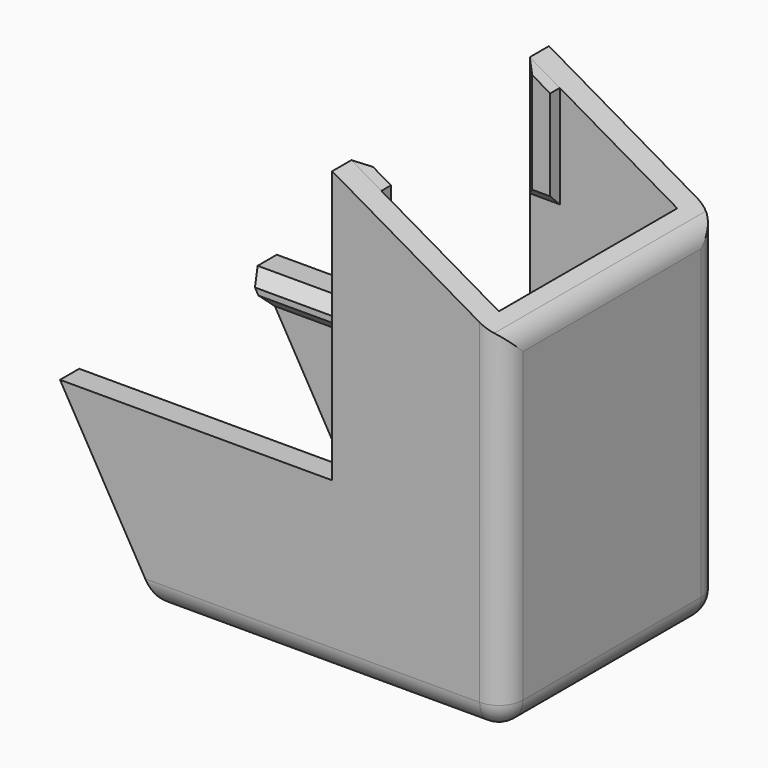
from build123d import *

# Parameters (mm, degrees)
F4_W      = 35
F4_H      = 18.6
F5_DEPTH  = 2
F4_W_2    = 2
F4_H_2    = 2
F6_DEPTH  = 37
F7_DEPTH  = 14.3
F8_W      = 2
F8_H      = 22.7
F9_DEPTH  = 12.3
F11_DEPTH = 22.6
F12_R     = 2
F14_DEPTH = 1
F15_SIZE  = 0.99999
F17_DEPTH = 1
F18_SIZE  = 0.99999


# Not quite as in the source:
# - a fillet or chamfer is up to 0.001 mm smaller than in the source, because OpenCascade refuses the exact size


with BuildPart() as f5:
    # F4 (on Top) → F5 (new body)
    with BuildSketch(Plane.XY):
        with Locations((17.5, -11.3)):
            Rectangle(F4_W, F4_H)
    extrude(amount=F5_DEPTH)

    # F4 (on Top) → F6 (join)
    with BuildSketch(Plane.XY):
        with Locations((36, -11.3)):
            Rectangle(F4_W_2, F4_H)
        with Locations((36, -21.6)):
            Rectangle(F4_W_2, F4_H_2)
        with Locations((36, -1)):
            Rectangle(F4_W_2, F4_H_2)
    extrude(amount=F6_DEPTH)

    # F4 (on Top) → F7 (join)
    with BuildSketch(Plane.XY):
        with Locations((17.5, -1)):
            Rectangle(F4_W, F4_H_2)
        with Locations((17.5, -21.6)):
            Rectangle(F4_W, F4_H_2)
    extrude(amount=F7_DEPTH)

    # F8 (on face) → F9 (join)
    with BuildSketch(Plane(origin=(35, 0, 0), x_dir=(0, -1, 0), z_dir=(-1, 0, 0))):
        with Locations((1, 25.65)):
            Rectangle(F8_W, F8_H)
        with Locations((21.6, 25.65)):
            Rectangle(F8_W, F8_H)
    extrude(amount=F9_DEPTH)

    # F10 (on face) → F11 (cut)
    with BuildSketch(Plane.XZ.offset(22.6)):
        Polygon((8.2561088494, 0), (0, 14.3), (0, 0), align=None)
        Polygon((37, 37), (22.7, 37), (37, 28.7438911506), align=None)
    extrude(amount=-F11_DEPTH, mode=Mode.SUBTRACT)

    # F12
    f12_edges = [f5.edges().sort_by_distance(p)[0] for p in [
        (37, -11.3, 0),
        (22.628054, -22.6, 0),
        (37, -22.6, 14.371946),
        (37, 0, 14.371946),
        (22.628054, 0, 0),
        (8.256109, -11.3, 0),
        (37, -11.3, 28.743891),
    ]]
    fillet(f12_edges, radius=F12_R)

    # F13 (on face) → F14 (join)
    with BuildSketch(Plane.XZ.offset(2)):
        Polygon((25.2, 35.556624327), (22.7, 37), (22.7, 27), (25.2, 27), align=None)
        Polygon((10, 11.8), (10, 14.3), (0, 14.3), (1.443375673, 11.8), align=None)
    extrude(amount=F14_DEPTH)

    # F15 (size 1 in the source; OpenCascade refuses exactly that, so slightly less here)
    f15_edges = [f5.edges().sort_by_distance(p)[0] for p in [
        (23.95, -3, 27),
        (5.721688, -3, 11.8),
        (22.7, -3, 32),
        (5, -3, 14.3),
    ]]
    chamfer(f15_edges, length=F15_SIZE)

    # F16 (on face) → F17 (join)
    with BuildSketch(Plane(origin=(0, -20.6, 0), x_dir=(-1, 0, 0), z_dir=(0, 1, 0))):
        Polygon((-22.7, 27), (-22.7, 37), (-25.2, 35.556624327), (-25.2, 27), align=None)
        Polygon((0, 14.3), (-10, 14.3), (-10, 11.8), (-1.443375673, 11.8), align=None)
    extrude(amount=F17_DEPTH)

    # F18 (size 1 in the source; OpenCascade refuses exactly that, so slightly less here)
    f18_edges = [f5.edges().sort_by_distance(p)[0] for p in [
        (5.721688, -19.6, 11.8),
        (5, -19.6, 14.3),
        (22.7, -19.6, 32),
        (23.95, -19.6, 27),
    ]]
    chamfer(f18_edges, length=F18_SIZE)


solid = f5.part
